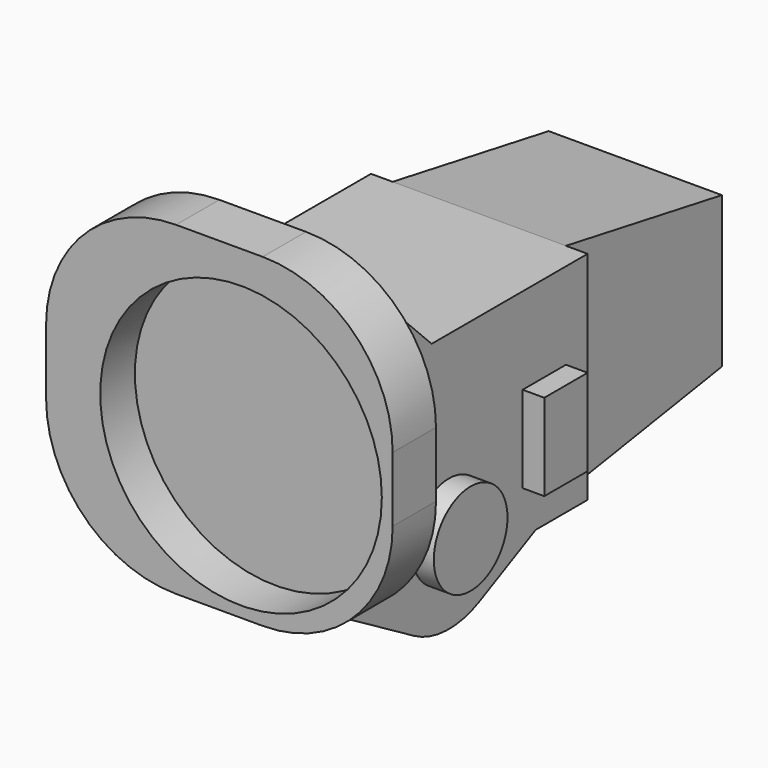
from build123d import *

# Parameters (mm, degrees)
F1_DEPTH      = 203.2
F1_DEPTH_BACK = 203.2
F0_W          = 63.5
F0_H          = 101.6
F0_R          = 54
F2_DEPTH      = 127
F2_DEPTH_BACK = 127
F3_DEPTH      = 101.6
F3_DEPTH_BACK = 101.6
F4_DEPTH      = 152.4
F4_DEPTH_BACK = 114.3
F5_T1_DEPTH   = 825.5
F5_T6_DEPTH   = 825.5
F5_T11_DEPTH  = 444.5
F5_T16_DEPTH  = 825.5
F5_T21_DEPTH  = 825.5
F6_DEPTH      = 152.4
F6_DEPTH_BACK = 152.4
F7_R          = 165.1
F8_DEPTH      = 50.8


# Not quite as in the source:
# - a fillet or chamfer that OpenCascade refuses, or shapes differently, is made with other operations: its cross-section is extruded or revolved along the edge and cut away or added


with BuildPart() as f1:
    # F0 (on Right) → F1 (new body, two sides)
    with BuildSketch(Plane.YZ) as f1_sk:
        Polygon((-177.8, -50.8), (-114.3, -50.8), (-114.3, 292.1), (-114.3, 330.2), (-177.8, 330.2), align=None)
    extrude(amount=F1_DEPTH)
    extrude(f1_sk.sketch, amount=-F1_DEPTH_BACK)

    # F0 (on Right) → F2 (join, two sides)
    with BuildSketch(Plane.YZ) as f2_sk:
        with BuildLine():
            ThreePointArc((-51.3464921696, -87.6703926185), (-50.5260150594, 88.1457985511), (101.6, 0))
            ThreePointArc((101.6, 0), (86.2402819365, -53.7138136006), (44.8052407181, -91.1868982047))
            Line((44.8052407181, -91.1868982047), (127, -50.8))
            Line((127, -50.8), (203.2, -50.8))
            Line((203.2, -50.8), (203.2, 203.2))
            Line((203.2, 203.2), (-25.4, 203.2))
            Line((-25.4, 203.2), (-114.3, 292.1))
            Line((-114.3, 292.1), (-114.3, -50.8))
            Line((-114.3, -50.8), (-51.3464921696, -87.6703926185))
        make_face()
        with Locations((139.7, 50.8)):
            Rectangle(F0_W, F0_H, mode=Mode.SUBTRACT)
        with BuildLine():
            ThreePointArc((44.8052407181, -91.1868982047), (86.2402819365, -53.7138136006), (101.6, 0))
            ThreePointArc((101.6, 0), (-50.5260150594, 88.1457985511), (-51.3464921696, -87.6703926185))
            ThreePointArc((-51.3464921696, -87.6703926185), (-3.7132796181, -101.5321208016), (44.8052407181, -91.1868982047))
        make_face()
        Circle(F0_R, mode=Mode.SUBTRACT)
    extrude(amount=F2_DEPTH)
    extrude(f2_sk.sketch, amount=-F2_DEPTH_BACK)

    # F0 (on Right) → F3 (join, two sides)
    with BuildSketch(Plane.YZ) as f3_sk:
        Polygon((203.2, 203.2), (203.2, -50.8), (431.8, -14.3826426938), (431.8, 162.6118868589), align=None)
    extrude(amount=F3_DEPTH)
    extrude(f3_sk.sketch, amount=-F3_DEPTH_BACK)

    # F0 (on Right) → F4 (join, two sides)
    with BuildSketch(Plane.YZ) as f4_sk:
        Circle(F0_R)
    extrude(amount=F4_DEPTH)
    extrude(f4_sk.sketch, amount=-F4_DEPTH_BACK)

    # F5: fillet of radius 152.4 on 4 edges, made by hand

    # F5_s2 → F5_t1 (cut)
    with BuildSketch(Plane.XZ.offset(-266.7)):
        with BuildLine():
            ThreePointArc((203.2, 177.8), (158.5630734528, 285.5630734528), (50.8, 330.2))
            Line((50.8, 330.2), (203.2, 330.2))
            Line((203.2, 330.2), (203.2, 177.8))
        make_face()
        with BuildLine():
            ThreePointArc((-203.2, 177.8), (-158.5630734528, 285.5630734528), (-50.8, 330.2))
            Line((-50.8, 330.2), (-203.2, 330.2))
            Line((-203.2, 330.2), (-203.2, 177.8))
        make_face()
    extrude(amount=F5_T1_DEPTH, mode=Mode.SUBTRACT)


with BuildPart() as f5_tool4:
    # F5_s5 → F5_t6 (new body)
    with BuildSketch(Plane.XZ.offset(558.8)):
        with BuildLine():
            ThreePointArc((50.8, -50.8), (158.5630734528, -6.1630734528), (203.2, 101.6))
            Line((203.2, 101.6), (203.2, -50.8))
            Line((203.2, -50.8), (50.8, -50.8))
        make_face()
    extrude(amount=-F5_T6_DEPTH)

    split(bisect_by=Plane(origin=(0, -51.3464921696, -87.6703926185), x_dir=(1, 0, 0), z_dir=(0, -0.5053788599, -0.8628975651)), keep=Keep.TOP)


with BuildPart() as f1_1:
    add(f1.part)

    # F5_t3: cut F5_tool4
    add(f5_tool4.part, mode=Mode.SUBTRACT)


with BuildPart() as f5_tool9:
    # F5_s10 → F5_t11 (new body)
    with BuildSketch(Plane.XZ.offset(558.8)):
        with BuildLine():
            ThreePointArc((50.8, -50.8), (158.5630734528, -6.1630734528), (203.2, 101.6))
            Line((203.2, 101.6), (203.2, -50.8))
            Line((203.2, -50.8), (50.8, -50.8))
        make_face()
    extrude(amount=-F5_T11_DEPTH)

    split(bisect_by=Plane.YZ.offset(127), keep=Keep.TOP)


with BuildPart() as f1_2:
    add(f1_1.part)

    # F5_t8: cut F5_tool9
    add(f5_tool9.part, mode=Mode.SUBTRACT)


with BuildPart() as f5_tool14:
    # F5_s15 → F5_t16 (new body)
    with BuildSketch(Plane.XZ.offset(558.8)):
        with BuildLine():
            ThreePointArc((-50.8, -50.8), (-158.5630734528, -6.1630734528), (-203.2, 101.6))
            Line((-203.2, 101.6), (-203.2, -50.8))
            Line((-203.2, -50.8), (-50.8, -50.8))
        make_face()
    extrude(amount=-F5_T16_DEPTH)

    split(bisect_by=Plane(origin=(0, -51.3464921696, -87.6703926185), x_dir=(1, 0, 0), z_dir=(0, -0.5053788599, -0.8628975651)), keep=Keep.TOP)


with BuildPart() as f1_3:
    add(f1_2.part)

    # F5_t13: cut F5_tool14
    add(f5_tool14.part, mode=Mode.SUBTRACT)


with BuildPart() as f5_tool19:
    # F5_s20 → F5_t21 (new body)
    with BuildSketch(Plane.XZ.offset(558.8)):
        with BuildLine():
            ThreePointArc((-50.8, -50.8), (-158.5630734528, -6.1630734528), (-203.2, 101.6))
            Line((-203.2, 101.6), (-203.2, -50.8))
            Line((-203.2, -50.8), (-50.8, -50.8))
        make_face()
    extrude(amount=-F5_T21_DEPTH)

    split(bisect_by=Plane.YZ.offset(-127), keep=Keep.BOTTOM)


with BuildPart() as f1_4:
    add(f1_3.part)

    # F5_t18: cut F5_tool19
    add(f5_tool19.part, mode=Mode.SUBTRACT)

    # F0 (on Right) → F6 (join, two sides)
    with BuildSketch(Plane.YZ) as f6_sk:
        with Locations((139.7, 50.8)):
            Rectangle(F0_W, F0_H)
    extrude(amount=F6_DEPTH)
    extrude(f6_sk.sketch, amount=-F6_DEPTH_BACK)

    # F7 (on face) → F8 (cut)
    with BuildSketch(Plane.XZ.offset(177.8)):
        with Locations((25.4, 127)):
            Circle(F7_R)
    extrude(amount=-F8_DEPTH, mode=Mode.SUBTRACT)


solid = f1_4.part
